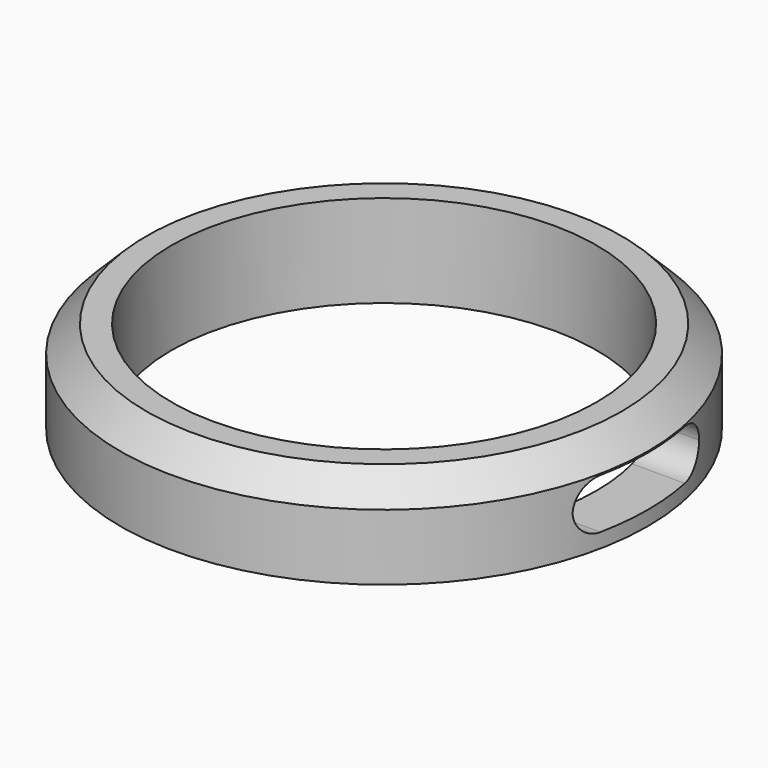
from build123d import *

# Parameters (mm, degrees)
F0_R         = 10
F0_R_2       = 8.05
F1_DEPTH     = 3.5
F3_DEPTH     = 16.9
F4_T4_DEPTH  = 7.0692849199
F4_S5_R      = 10
F4_T6_DEPTH  = 5
F4_S7_R      = 8.05
F4_T8_DEPTH  = 5
F4_T12_DEPTH = 7.0692849199
F4_S13_R     = 10
F4_T14_DEPTH = 5
F4_S15_R     = 8.05
F4_T16_DEPTH = 5
F4_T20_DEPTH = 7.0692849199
F4_S21_R     = 10
F4_T22_DEPTH = 5
F4_S23_R     = 8.05
F4_T24_DEPTH = 5
F4_T28_DEPTH = 7.0692849199
F4_S29_R     = 10
F4_T30_DEPTH = 5
F4_S31_R     = 8.05
F4_T32_DEPTH = 5
F5_SIZE      = 1


# Not quite as in the source:
# - a fillet or chamfer that OpenCascade refuses, or shapes differently, is made with other operations: its cross-section is extruded or revolved along the edge and cut away or added


with BuildPart() as f1:
    # F0 (on Top) → F1 (new body)
    with BuildSketch(Plane.XY):
        Circle(F0_R)
        Circle(F0_R_2, mode=Mode.SUBTRACT)
    extrude(amount=F1_DEPTH)

    # F2 (on Right) → F3 (cut)
    with BuildSketch(Plane.YZ):
        Polygon((3, 0.55), (3, 2.45), (-3, 2.45), (-3, 0.55), (0, 0.55), align=None)
    extrude(amount=F3_DEPTH, mode=Mode.SUBTRACT)

    # F4: fillet of radius 1 on 4 edges, made by hand


with BuildPart() as f4_tool2:
    # F4_s3 → F4_t4 (new body)
    with BuildSketch(Plane.YZ.offset(4.9701070943)):
        with BuildLine():
            ThreePointArc((2, 2.45), (2.7071067812, 2.1571067812), (3, 1.45))
            Line((3, 1.45), (3, 2.45))
            Line((3, 2.45), (2, 2.45))
        make_face()
    extrude(amount=F4_T4_DEPTH)

    # F4_s5 → F4_t6 (intersect, symmetric)
    with BuildSketch(Plane.XY.offset(2)):
        Circle(F4_S5_R)
    extrude(amount=F4_T6_DEPTH, both=True, mode=Mode.INTERSECT)

    # F4_s7 → F4_t8 (cut, symmetric)
    with BuildSketch(Plane.XY.offset(2)):
        Circle(F4_S7_R)
    extrude(amount=F4_T8_DEPTH, both=True, mode=Mode.SUBTRACT)


with BuildPart() as f1_1:
    add(f1.part)

    # F4_t1: union F4_tool2
    add(f4_tool2.part)


with BuildPart() as f4_tool10:
    # F4_s11 → F4_t12 (new body)
    with BuildSketch(Plane.YZ.offset(4.9701070943)):
        with BuildLine():
            ThreePointArc((2, 0.55), (2.7071067812, 0.8428932188), (3, 1.55))
            Line((3, 1.55), (3, 0.55))
            Line((3, 0.55), (2, 0.55))
        make_face()
    extrude(amount=F4_T12_DEPTH)

    # F4_s13 → F4_t14 (intersect, symmetric)
    with BuildSketch(Plane.XY.offset(1.1)):
        Circle(F4_S13_R)
    extrude(amount=F4_T14_DEPTH, both=True, mode=Mode.INTERSECT)

    # F4_s15 → F4_t16 (cut, symmetric)
    with BuildSketch(Plane.XY.offset(1.1)):
        Circle(F4_S15_R)
    extrude(amount=F4_T16_DEPTH, both=True, mode=Mode.SUBTRACT)


with BuildPart() as f1_2:
    add(f1_1.part)

    # F4_t9: union F4_tool10
    add(f4_tool10.part)


with BuildPart() as f4_tool18:
    # F4_s19 → F4_t20 (new body)
    with BuildSketch(Plane.YZ.offset(4.9701070943)):
        with BuildLine():
            ThreePointArc((-3, 1.45), (-2.7071067812, 2.1571067812), (-2, 2.45))
            Line((-2, 2.45), (-3, 2.45))
            Line((-3, 2.45), (-3, 1.45))
        make_face()
    extrude(amount=F4_T20_DEPTH)

    # F4_s21 → F4_t22 (intersect, symmetric)
    with BuildSketch(Plane.XY.offset(2)):
        Circle(F4_S21_R)
    extrude(amount=F4_T22_DEPTH, both=True, mode=Mode.INTERSECT)

    # F4_s23 → F4_t24 (cut, symmetric)
    with BuildSketch(Plane.XY.offset(2)):
        Circle(F4_S23_R)
    extrude(amount=F4_T24_DEPTH, both=True, mode=Mode.SUBTRACT)


with BuildPart() as f1_3:
    add(f1_2.part)

    # F4_t17: union F4_tool18
    add(f4_tool18.part)


with BuildPart() as f4_tool26:
    # F4_s27 → F4_t28 (new body)
    with BuildSketch(Plane.YZ.offset(4.9701070943)):
        with BuildLine():
            ThreePointArc((-2, 0.55), (-2.7071067812, 0.8428932188), (-3, 1.55))
            Line((-3, 1.55), (-3, 0.55))
            Line((-3, 0.55), (-2, 0.55))
        make_face()
    extrude(amount=F4_T28_DEPTH)

    # F4_s29 → F4_t30 (intersect, symmetric)
    with BuildSketch(Plane.XY.offset(1.1)):
        Circle(F4_S29_R)
    extrude(amount=F4_T30_DEPTH, both=True, mode=Mode.INTERSECT)

    # F4_s31 → F4_t32 (cut, symmetric)
    with BuildSketch(Plane.XY.offset(1.1)):
        Circle(F4_S31_R)
    extrude(amount=F4_T32_DEPTH, both=True, mode=Mode.SUBTRACT)


with BuildPart() as f1_4:
    add(f1_3.part)

    # F4_t25: union F4_tool26
    add(f4_tool26.part)

    # F5
    f5_edges = [f1_4.edges().sort_by_distance(p)[0] for p in [
        (-10, 0, 3.5),
    ]]
    chamfer(f5_edges, length=F5_SIZE)


solid = f1_4.part
